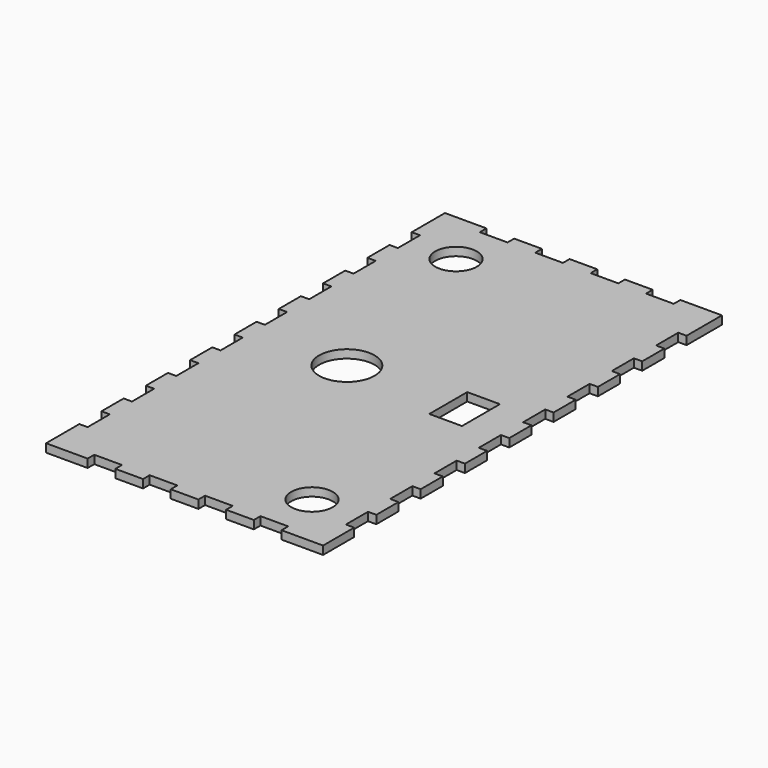
from build123d import *

# Parameters (mm, degrees)
F0_R     = 10
F0_R_2   = 7.5
F0_W     = 11.8
F0_H     = 17.1
F1_DEPTH = 1.5


# Not quite as in the source:
# - ends of sketch curves that miss each other by under 0.0002 mm in the source are joined


with BuildPart() as f1:
    # F0 (on Top) → F1 (new body, symmetric)
    with BuildSketch(Plane.XY):
        Polygon((-46.9999983907, 3.8743e-06), (-46.9999983907, -4.9999961257), (-43.9999983907, -4.9999961257), (-43.9999983907, -14.9999961257), (-46.9999983907, -14.9999961257), (-46.9999983907, -24.9999961257), (-43.9999983907, -24.9999961257), (-43.9999983907, -34.9999961257), (-46.9999983907, -34.9999961257), (-46.9999983907, -44.9999961257), (-43.9999983907, -44.9999961257), (-43.9999983907, -54.9999961257), (-46.9999983907, -54.9999961257), (-46.9999983907, -64.9999961257), (-43.9999983907, -64.9999961257), (-43.9999983907, -74.9999961257), (-46.9999983907, -74.9999961257), (-46.9999983907, -89.9999961257), (-31.9999983907, -89.9999961257), (-31.9999983907, -86.9999961257), (-21.9999983907, -86.9999961257), (-21.9999983907, -89.9999961257), (-11.9999983907, -89.9999961257), (-11.9999983907, -86.9999961257), (-1.9999983907, -86.9999961257), (-1.9999983907, -89.9999961257), (8.0000016093, -89.9999961257), (8.0000016093, -86.9999961257), (18.0000016093, -86.9999961257), (18.0000016093, -89.9999961257), (28.0000016093, -89.9999961257), (28.0000016093, -86.9999961257), (38.0000016093, -86.9999961257), (38.0000016093, -89.9999961257), (53.0000016093, -89.9999961257), (53.0000030994, -75.968132019), (50.0000030994, -75.968132019), (50.0000030994, -65.968132019), (53.0000030994, -65.968132019), (53.0000030994, -55.968132019), (50.0000030994, -55.968132019), (50.0000030994, -45.968132019), (53.0000030994, -45.968132019), (53.0000030994, -35.968132019), (50.0000030994, -35.968132019), (50.0000030994, -25.968132019), (53.0000030994, -25.968132019), (53.0000030994, -15.968132019), (50.0000030994, -15.968132019), (50.0000030994, -5.968132019), (53.0000030994, -5.968132019), (53.0000030994, 3.8743e-06), (53.0000030994, 4.031867981), (50.0000030994, 4.031867981), (50.0000030994, 14.031867981), (53.0000030994, 14.031867981), (53.0000030994, 24.031867981), (50.0000030994, 24.031867981), (50.0000030994, 34.031867981), (53.0000030994, 34.031867981), (53.0000030994, 44.031867981), (50.0000030994, 44.031867981), (50.0000030994, 54.031867981), (53.0000030994, 54.031867981), (53.0000030994, 64.031867981), (50.0000030994, 64.031867981), (50.0000030994, 74.031867981), (53.0000030994, 74.031867981), (53.0000030994, 90.0000038743), (38.0000016093, 90.0000035763), (38.0000016093, 87.0000035763), (28.0000016093, 87.0000035763), (28.0000016093, 90.0000035763), (18.0000016093, 90.0000035763), (18.0000016093, 87.0000035763), (8.0000016093, 87.0000035763), (8.0000016093, 90.0000035763), (-1.9999983907, 90.0000035763), (-1.9999983907, 87.0000035763), (-11.9999983907, 87.0000035763), (-11.9999983907, 90.0000035763), (-21.9999983907, 90.0000035763), (-21.9999983907, 87.0000035763), (-31.9999983907, 87.0000035763), (-31.9999983907, 90.0000035763), (-46.9999983907, 90.0000035763), (-46.9999983907, 75.0000038743), (-43.9999983907, 75.0000038743), (-43.9999983907, 65.0000038743), (-46.9999983907, 65.0000038743), (-46.9999983907, 55.0000038743), (-43.9999983907, 55.0000038743), (-43.9999983907, 45.0000038743), (-46.9999983907, 45.0000038743), (-46.9999983907, 35.0000038743), (-43.9999983907, 35.0000038743), (-43.9999983907, 25.0000038743), (-46.9999983907, 25.0000038743), (-46.9999983907, 15.0000038743), (-43.9999983907, 15.0000038743), (-43.9999983907, 5.0000038743), (-46.9999983907, 5.0000038743), align=None)
        with Locations((-10.3999983907, 3.8743e-06)):
            Circle(F0_R, mode=Mode.SUBTRACT)
        with Locations((33.0000030994, -69.9999961257)):
            Circle(F0_R_2, mode=Mode.SUBTRACT)
        with Locations((-26.9999983907, 70.0000035763)):
            Circle(F0_R_2, mode=Mode.SUBTRACT)
        with Locations((32.1000030994, 3.8743e-06)):
            Rectangle(F0_W, F0_H, mode=Mode.SUBTRACT)
    extrude(amount=F1_DEPTH, both=True)


solid = f1.part
